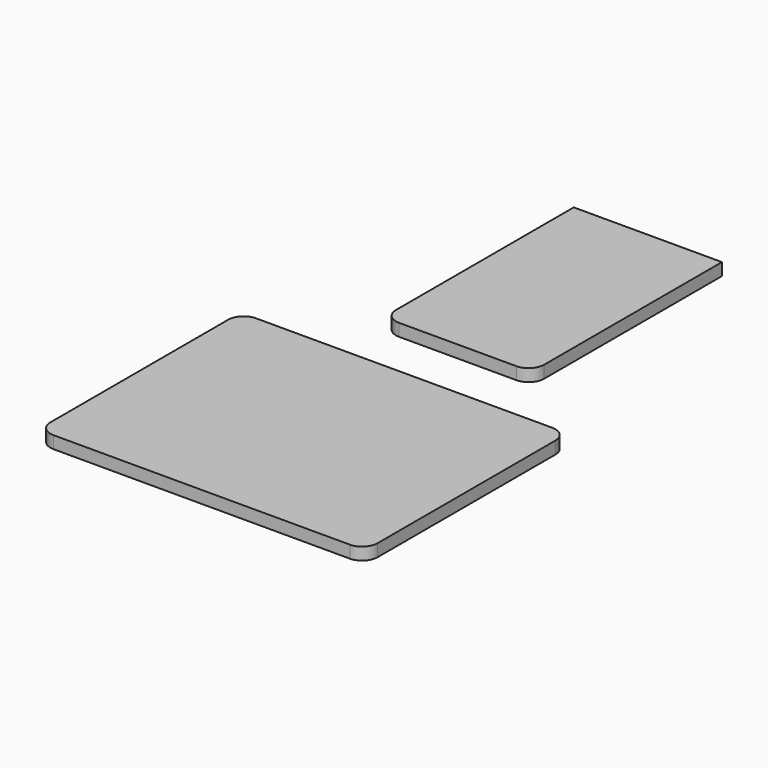
from build123d import *

# Parameters (mm, degrees)
F0_W     = 106
F0_H     = 82
F2_DEPTH = 4
F3_R     = 5
F3_2_R   = 5


# Not quite as in the source:
# - a feature names something its author has since deleted; it is built from what else it names


with BuildPart() as f2:
    # F0 (on Top) → F2 (new body)
    with BuildSketch(Plane.XY):
        with Locations((0, -43.5)):
            Rectangle(F0_W, F0_H)
    extrude(amount=F2_DEPTH)

    # F3
    f3_edges = [f2.edges().sort_by_distance(p)[0] for p in [
        (53, -84.5, 2),
        (-53, -84.5, 2),
        (-53, -2.5, 2),
        (53, -2.5, 2),
    ]]
    fillet(f3_edges, radius=F3_R)


with BuildPart() as f2b:
    # F1 (on Top) → F2, piece 2 (new body)
    with BuildSketch(Plane.XY):
        Polygon((24.8151908007, 18.1759698881), (24.8151908007, 95.1759698881), (-23.1848091993, 95.1759698881), (-23.1848091993, 88.1759698881), (-23.1848091993, 18.1759698881), (-4.1848091993, 18.1759698881), (5.8151908007, 18.1759698881), align=None)
    extrude(amount=F2_DEPTH)

    # F3#2
    f3_2_edges = [f2b.edges().sort_by_distance(p)[0] for p in [
        (-23.184809, 18.17597, 2),
        (24.815191, 18.17597, 2),
    ]]
    fillet(f3_2_edges, radius=F3_2_R)


solid = Compound([f2.part, f2b.part])
